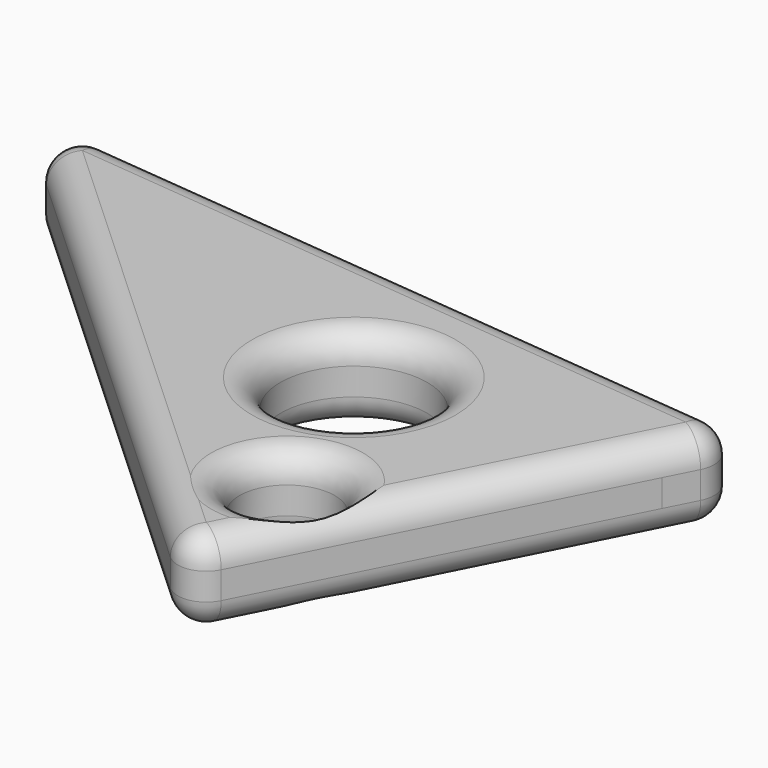
from build123d import *

# Parameters (mm, degrees)
F0_R         = 14.451692169
F0_R_2       = 22.2877793756
F1_DEPTH     = 25.4
F2_T1_DEPTH  = 199.3743361021
F2_T3_DEPTH  = 192.7884894302
F2_T5_DEPTH  = 8.2301131444
F2_T7_DEPTH  = 124.5333156844
F2_T12_DEPTH = 8.5849434278
F2_T18_DEPTH = 8.5849434278
F2_T24_DEPTH = 8.5849434278
F2_T30_DEPTH = 8.5849434278
F2_T36_DEPTH = 8.5849434278
F2_T42_DEPTH = 8.5849434278


# Not quite as in the source:
# - a fillet or chamfer that OpenCascade refuses, or shapes differently, is made with other operations: its cross-section is extruded or revolved along the edge and cut away or added


with BuildPart() as f1:
    # F0 (on Top) → F1 (new body)
    with BuildSketch(Plane.XY):
        with BuildLine():
            Line((-113.832257688, 69.7422921658), (55.3128607571, -85.7750177383))
            Line((55.3128607571, -85.7750177383), (98.9801470389, 0))
            ThreePointArc((98.9801470389, 0), (88.9042904179, 21.7216579157), (112.3967300467, 26.3539996064))
            Line((112.3967300467, 26.3539996064), (122.6502582431, 46.4948564768))
            Line((122.6502582431, 46.4948564768), (4.4090002775, 58.1185743213))
            ThreePointArc((4.4090002775, 58.1185743213), (-12.006964874, 45.4296421416), (-25.6377878195, 61.0723266154))
            Line((-25.6377878195, 61.0723266154), (-77.869777953, 66.2069972558))
            ThreePointArc((-77.869777953, 66.2069972558), (-87.4993555937, 58.3520393661), (-95.4150132583, 67.9317832418))
            Line((-95.4150132583, 67.9317832418), (-113.832257688, 69.7422921658))
        make_face()
        with Locations((54.5112267137, -43.2883314788)):
            Circle(F0_R, mode=Mode.SUBTRACT)
        with Locations((33.6687006056, 8.0163478851)):
            Circle(F0_R_2, mode=Mode.SUBTRACT)
        with BuildLine():
            ThreePointArc((112.3967300467, 26.3539996064), (88.9042904179, 21.7216579157), (98.9801470389, 0))
            Line((98.9801470389, 0), (112.3967300467, 26.3539996064))
        make_face()
        with BuildLine():
            Line((-77.869777953, 66.2069972558), (-95.4150132583, 67.9317832418))
            ThreePointArc((-95.4150132583, 67.9317832418), (-87.4993555937, 58.3520393661), (-77.869777953, 66.2069972558))
        make_face()
        with BuildLine():
            ThreePointArc((-25.6377878195, 61.0723266154), (-12.006964874, 45.4296421416), (4.4090002775, 58.1185743213))
            Line((4.4090002775, 58.1185743213), (-25.6377878195, 61.0723266154))
        make_face()
    extrude(amount=F1_DEPTH)

    # F2: fillet of radius 8.5849434278 on 15 edges, made by hand

    # F2_s2 → F2_t1 (cut)
    with BuildSketch(Plane(origin=(104.4327323095, -10.2662694476, 0), x_dir=(0, 0, 1), z_dir=(-0.9952027962, 0.0978335033, 0))):
        with BuildLine():
            ThreePointArc((16.8150565722, 58.2711156209), (22.8855282861, 55.756643907), (25.4, 49.6861721931))
            Line((25.4, 49.6861721931), (25.4, 58.2711156209))
            Line((25.4, 58.2711156209), (16.8150565722, 58.2711156209))
        make_face()
        with BuildLine():
            ThreePointArc((8.5849434278, 58.2711156209), (2.5144717139, 55.756643907), (0, 49.6861721931))
            Line((0, 49.6861721931), (0, 58.2711156209))
            Line((0, 58.2711156209), (8.5849434278, 58.2711156209))
        make_face()
    extrude(amount=F2_T1_DEPTH, mode=Mode.SUBTRACT)

    # F2_s4 → F2_t3 (cut)
    with BuildSketch(Plane(origin=(-77.5368310442, 71.289786506, 0), x_dir=(0, 0, 1), z_dir=(0.7361395861, -0.6768297495, 0))):
        with BuildLine():
            ThreePointArc((16.8150565722, 25.7049963658), (22.8855282861, 23.1905246519), (25.4, 17.120052938))
            Line((25.4, 17.120052938), (25.4, 25.7049963658))
            Line((25.4, 25.7049963658), (16.8150565722, 25.7049963658))
        make_face()
        with BuildLine():
            ThreePointArc((8.5849434278, 25.7049963658), (2.5144717139, 23.1905246519), (0, 17.120052938))
            Line((0, 17.120052938), (0, 25.7049963658))
            Line((0, 25.7049963658), (8.5849434278, 25.7049963658))
        make_face()
    extrude(amount=F2_T3_DEPTH, mode=Mode.SUBTRACT)

    # F2_s6 → F2_t5 (cut)
    with BuildSketch(Plane.XY.offset(8.5849434278)):
        with BuildLine():
            ThreePointArc((-94.9347372949, 52.3673211207), (-96.9604906178, 62.1932723461), (-88.2842970942, 67.2307975271))
            Line((-88.2842970942, 67.2307975271), (-113.832257688, 69.7422921658))
            Line((-113.832257688, 69.7422921658), (-94.9347372949, 52.3673211207))
        make_face()
        with BuildLine():
            ThreePointArc((46.9845015181, -78.1176638834), (54.3170318204, -80.2469006514), (60.4456313968, -75.6927907406))
            Line((60.4456313968, -75.6927907406), (55.3128607571, -85.7750177383))
            Line((55.3128607571, -85.7750177383), (46.9845015181, -78.1176638834))
        make_face()
        with BuildLine():
            ThreePointArc((116.94428937, 35.2867044944), (116.8237626916, 43.3045904742), (110.1335996919, 47.725307758))
            Line((110.1335996919, 47.725307758), (122.6502582431, 46.4948564768))
            Line((122.6502582431, 46.4948564768), (116.94428937, 35.2867044944))
        make_face()
    extrude(amount=F2_T5_DEPTH, mode=Mode.SUBTRACT)

    # F2_s8 → F2_t7 (cut)
    with BuildSketch(Plane(origin=(-18.161596753, -35.6745613546, 0), x_dir=(0, 0, 1), z_dir=(0.453683078, 0.8911630966, 0))):
        with BuildLine():
            ThreePointArc((8.5849434278, 88.2074543369), (2.5144717139, 85.692982623), (0, 79.6225109091))
            Line((0, 79.6225109091), (0, 88.2074543369))
            Line((0, 88.2074543369), (8.5849434278, 88.2074543369))
        make_face()
        with BuildLine():
            ThreePointArc((16.8150565722, 88.2074543369), (22.8855282861, 85.692982623), (25.4, 79.6225109091))
            Line((25.4, 79.6225109091), (25.4, 88.2074543369))
            Line((25.4, 88.2074543369), (16.8150565722, 88.2074543369))
        make_face()
    extrude(amount=F2_T7_DEPTH, mode=Mode.SUBTRACT)


with BuildPart() as f2_tool10:
    # F2_s11 → F2_t12 (new body)
    with BuildSketch(Plane.XY.offset(16.8150565722)):
        Polygon((109.2937046007, 39.1815480531), (116.94428937, 35.2867044944), (122.6502582431, 46.4948564768), (110.1335996919, 47.725307758), align=None)
    extrude(amount=F2_T12_DEPTH)

    # F2_s13 → F2_t14 (revolve, cut)
    with BuildSketch(Plane(origin=(109.2937046007, 39.1815480531, 16.8150565722), x_dir=(-0.877123787, -0.480264367, 0), z_dir=(-0.480264367, 0.877123787, 0))):
        with BuildLine():
            ThreePointArc((0, -8.5849434278), (8.5849434278, 0), (0, 8.5849434278))
            Line((0, 8.5849434278), (0, -8.5849434278))
        make_face()
    revolve(axis=Axis((109.2937046007, 39.1815480531, 16.8150565722), (0, 0, 1)), mode=Mode.SUBTRACT)


with BuildPart() as f1_1:
    add(f1.part)

    # F2_t9: cut F2_tool10
    add(f2_tool10.part, mode=Mode.SUBTRACT)


with BuildPart() as f2_tool16:
    # F2_s17 → F2_t18 (new body)
    with BuildSketch(Plane.XY.offset(16.8150565722)):
        Polygon((-89.1241921853, 58.6870378223), (-94.9347372949, 52.3673211207), (-113.832257688, 69.7422921658), (-88.2842970942, 67.2307975271), align=None)
    extrude(amount=F2_T18_DEPTH)

    # F2_s19 → F2_t20 (revolve, cut)
    with BuildSketch(Plane(origin=(-89.1241921853, 58.6870378223, 16.8150565722), x_dir=(0.912795582, -0.4084167302, 0), z_dir=(-0.4084167302, -0.912795582, 0))):
        with BuildLine():
            ThreePointArc((0, -8.5849434278), (8.5849434278, 0), (0, 8.5849434278))
            Line((0, 8.5849434278), (0, -8.5849434278))
        make_face()
    revolve(axis=Axis((-89.1241921853, 58.6870378223, 16.8150565722), (0, 0, 1)), mode=Mode.SUBTRACT)


with BuildPart() as f1_2:
    add(f1_1.part)

    # F2_t15: cut F2_tool16
    add(f2_tool16.part, mode=Mode.SUBTRACT)


with BuildPart() as f2_tool22:
    # F2_s23 → F2_t24 (new body)
    with BuildSketch(Plane.XY.offset(16.8150565722)):
        Polygon((52.7950466276, -71.7979471818), (46.9845015181, -78.1176638834), (55.3128607571, -85.7750177383), (60.4456313968, -75.6927907406), align=None)
    extrude(amount=F2_T24_DEPTH)

    # F2_s25 → F2_t26 (revolve, cut)
    with BuildSketch(Plane(origin=(52.7950466276, -71.7979471818, 16.8150565722), x_dir=(-0.1772854074, 0.9841594811, 0), z_dir=(0.9841594811, 0.1772854074, 0))):
        with BuildLine():
            ThreePointArc((0, -8.5849434278), (8.5849434278, 0), (0, 8.5849434278))
            Line((0, 8.5849434278), (0, -8.5849434278))
        make_face()
    revolve(axis=Axis((52.7950466276, -71.7979471818, 16.8150565722), (0, 0, 1)), mode=Mode.SUBTRACT)


with BuildPart() as f1_3:
    add(f1_2.part)

    # F2_t21: cut F2_tool22
    add(f2_tool22.part, mode=Mode.SUBTRACT)


with BuildPart() as f2_tool28:
    # F2_s29 → F2_t30 (new body)
    with BuildSketch(Plane.XY.offset(8.5849434278)):
        Polygon((-89.1241921853, 58.6870378223), (-94.9347372949, 52.3673211207), (-113.832257688, 69.7422921658), (-88.2842970942, 67.2307975271), align=None)
    extrude(amount=-F2_T30_DEPTH)

    # F2_s31 → F2_t32 (revolve, cut)
    with BuildSketch(Plane(origin=(-89.1241921853, 58.6870378223, 8.5849434278), x_dir=(0.912795582, -0.4084167302, 0), z_dir=(0.4084167302, 0.912795582, 0))):
        with BuildLine():
            ThreePointArc((0, -8.5849434278), (8.5849434278, 0), (0, 8.5849434278))
            Line((0, 8.5849434278), (0, -8.5849434278))
        make_face()
    revolve(axis=Axis((-89.1241921853, 58.6870378223, 8.5849434278), (0, 0, -1)), mode=Mode.SUBTRACT)


with BuildPart() as f1_4:
    add(f1_3.part)

    # F2_t27: cut F2_tool28
    add(f2_tool28.part, mode=Mode.SUBTRACT)


with BuildPart() as f2_tool34:
    # F2_s35 → F2_t36 (new body)
    with BuildSketch(Plane.XY.offset(8.5849434278)):
        Polygon((52.7950466276, -71.7979471818), (46.9845015181, -78.1176638834), (55.3128607571, -85.7750177383), (60.4456313968, -75.6927907406), align=None)
    extrude(amount=-F2_T36_DEPTH)

    # F2_s37 → F2_t38 (revolve, cut)
    with BuildSketch(Plane(origin=(52.7950466276, -71.7979471818, 8.5849434278), x_dir=(-0.1772854074, 0.9841594811, 0), z_dir=(-0.9841594811, -0.1772854074, 0))):
        with BuildLine():
            ThreePointArc((0, -8.5849434278), (8.5849434278, 0), (0, 8.5849434278))
            Line((0, 8.5849434278), (0, -8.5849434278))
        make_face()
    revolve(axis=Axis((52.7950466276, -71.7979471818, 8.5849434278), (0, 0, -1)), mode=Mode.SUBTRACT)


with BuildPart() as f1_5:
    add(f1_4.part)

    # F2_t33: cut F2_tool34
    add(f2_tool34.part, mode=Mode.SUBTRACT)


with BuildPart() as f2_tool40:
    # F2_s41 → F2_t42 (new body)
    with BuildSketch(Plane.XY.offset(8.5849434278)):
        Polygon((109.2937046007, 39.1815480531), (116.94428937, 35.2867044944), (122.6502582431, 46.4948564768), (110.1335996919, 47.725307758), align=None)
    extrude(amount=-F2_T42_DEPTH)

    # F2_s43 → F2_t44 (revolve, cut)
    with BuildSketch(Plane(origin=(109.2937046007, 39.1815480531, 8.5849434278), x_dir=(-0.877123787, -0.480264367, 0), z_dir=(0.480264367, -0.877123787, 0))):
        with BuildLine():
            ThreePointArc((0, -8.5849434278), (8.5849434278, 0), (0, 8.5849434278))
            Line((0, 8.5849434278), (0, -8.5849434278))
        make_face()
    revolve(axis=Axis((109.2937046007, 39.1815480531, 8.5849434278), (0, 0, -1)), mode=Mode.SUBTRACT)


with BuildPart() as f1_6:
    add(f1_5.part)

    # F2_t39: cut F2_tool40
    add(f2_tool40.part, mode=Mode.SUBTRACT)

    # F2_s45 → F2_t46 (revolve, cut)
    with BuildSketch(Plane.XZ.offset(43.2883314788)):
        with BuildLine():
            ThreePointArc((68.9629188827, 8.5849434278), (71.4773905966, 2.5144717139), (77.5478623105, 0))
            Line((77.5478623105, 0), (68.9629188827, 0))
            Line((68.9629188827, 0), (68.9629188827, 8.5849434278))
        make_face()
    revolve(axis=Axis((54.5112267137, -43.2883314788, 0), (0, 0, 1)), mode=Mode.SUBTRACT)

    # F2_s47 → F2_t48 (revolve, cut)
    with BuildSketch(Plane.XZ.offset(-8.0163478851)):
        with BuildLine():
            ThreePointArc((55.9564799812, 8.5849434278), (58.4709516951, 2.5144717139), (64.541423409, 0))
            Line((64.541423409, 0), (55.9564799812, 0))
            Line((55.9564799812, 0), (55.9564799812, 8.5849434278))
        make_face()
    revolve(axis=Axis((33.6687006056, 8.0163478851, 0), (0, 0, 1)), mode=Mode.SUBTRACT)

    # F2_s49 → F2_t50 (revolve, cut)
    with BuildSketch(Plane.XZ.offset(43.2883314788)):
        with BuildLine():
            ThreePointArc((68.9629188827, 16.8150565722), (71.4773905966, 22.8855282861), (77.5478623105, 25.4))
            Line((77.5478623105, 25.4), (68.9629188827, 25.4))
            Line((68.9629188827, 25.4), (68.9629188827, 16.8150565722))
        make_face()
    revolve(axis=Axis((54.5112267137, -43.2883314788, 25.4), (0, 0, 1)), mode=Mode.SUBTRACT)

    # F2_s51 → F2_t52 (revolve, cut)
    with BuildSketch(Plane.XZ.offset(-8.0163478851)):
        with BuildLine():
            ThreePointArc((55.9564799812, 16.8150565722), (58.4709516951, 22.8855282861), (64.541423409, 25.4))
            Line((64.541423409, 25.4), (55.9564799812, 25.4))
            Line((55.9564799812, 25.4), (55.9564799812, 16.8150565722))
        make_face()
    revolve(axis=Axis((33.6687006056, 8.0163478851, 25.4), (0, 0, 1)), mode=Mode.SUBTRACT)


solid = f1_6.part
